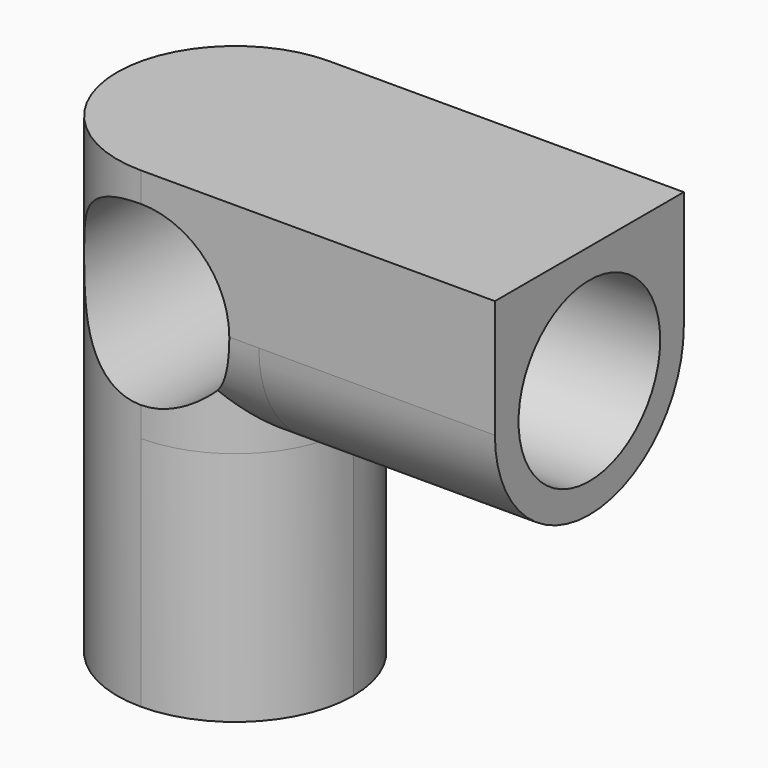
from build123d import *

# Parameters (mm, degrees)
F0_R         = 15
F1_DEPTH     = 40
F2_R         = 13
F3_DEPTH     = 40
F4_R         = 15
F5_DEPTH     = 40
F6_T3_DEPTH  = 40
F6_T6_DEPTH  = 40
F6_T9_DEPTH  = 80
F6_T12_DEPTH = 80
F6_T15_DEPTH = 40
F6_T18_DEPTH = 40
F6_T22_DEPTH = 90
F6_T26_DEPTH = 90
F6_T32_DEPTH = 90
F6_T36_DEPTH = 90


# Not quite as in the source:
# - a fillet or chamfer that OpenCascade refuses, or shapes differently, is made with other operations: its cross-section is extruded or revolved along the edge and cut away or added
# - a feature of the source that left no trace in its solid (it failed there, or was rolled back) is left out


with BuildPart() as f1:
    # F0 (on Front) → F1 (new body)
    with BuildSketch(Plane.XZ):
        Polygon((15, -40.7675257325), (15, -0.7675257325), (55, -0.7675257325), (55, 39.2324742675), (-25, 39.2324742675), (-25, -40.7675257325), align=None)
        with Locations((-5, 19.2324742675)):
            Circle(F0_R, mode=Mode.SUBTRACT)
    extrude(amount=F1_DEPTH)

    # F2 (on face) → F3 (cut)
    with BuildSketch(Plane(origin=(0, 0, -40.7675257325), x_dir=(1, 0, 0), z_dir=(0, 0, -1))):
        with Locations((-5, 20)):
            Circle(F2_R)
    extrude(amount=-F3_DEPTH, mode=Mode.SUBTRACT)

    # F4 (on face) → F5 (cut)
    with BuildSketch(Plane.YZ.offset(55)):
        with Locations((-20, 19.2324742675)):
            Circle(F4_R)
    extrude(amount=-F5_DEPTH, mode=Mode.SUBTRACT)

    # F6: fillet of radius 20 on 6 edges, made by hand


with BuildPart() as f6_tool1:
    # F6_s2 → F6_t3 (new body)
    with BuildSketch(Plane.XY.offset(-40.7675257325)):
        with BuildLine():
            ThreePointArc((-5, 0), (9.1421356237, -5.8578643763), (15, -20))
            Line((15, -20), (15.4, -20))
            Line((15.4, -20), (15.4, 0.4))
            Line((15.4, 0.4), (-5, 0.4))
            Line((-5, 0.4), (-5, 0))
        make_face()
    extrude(amount=F6_T3_DEPTH)


with BuildPart() as f6_tool4:
    # F6_s5 → F6_t6 (new body)
    with BuildSketch(Plane.XY.offset(-40.7675257325)):
        with BuildLine():
            ThreePointArc((-5, -40), (9.1421356237, -34.1421356237), (15, -20))
            Line((15, -20), (15.4, -20))
            Line((15.4, -20), (15.4, -40.4))
            Line((15.4, -40.4), (-5, -40.4))
            Line((-5, -40.4), (-5, -40))
        make_face()
    extrude(amount=F6_T6_DEPTH)


with BuildPart() as f6_tool7:
    # F6_s8 → F6_t9 (new body)
    with BuildSketch(Plane.XY.offset(39.2324742675)):
        with BuildLine():
            ThreePointArc((-25, -20), (-19.1421356237, -34.1421356237), (-5, -40))
            Line((-5, -40), (-5, -40.4))
            Line((-5, -40.4), (-25.4, -40.4))
            Line((-25.4, -40.4), (-25.4, -20))
            Line((-25.4, -20), (-25, -20))
        make_face()
    extrude(amount=-F6_T9_DEPTH)


with BuildPart() as f6_tool10:
    # F6_s11 → F6_t12 (new body)
    with BuildSketch(Plane.XY.offset(39.2324742675)):
        with BuildLine():
            ThreePointArc((-25, -20), (-19.1421356237, -5.8578643763), (-5, 0))
            Line((-5, 0), (-5, 0.4))
            Line((-5, 0.4), (-25.4, 0.4))
            Line((-25.4, 0.4), (-25.4, -20))
            Line((-25.4, -20), (-25, -20))
        make_face()
    extrude(amount=-F6_T12_DEPTH)


with BuildPart() as f6_tool13:
    # F6_s14 → F6_t15 (new body)
    with BuildSketch(Plane.YZ.offset(15)):
        with BuildLine():
            ThreePointArc((0, 19.2324742675), (-5.8578643763, 5.0903386438), (-20, -0.7675257325))
            Line((-20, -0.7675257325), (-20, -1.1675257325))
            Line((-20, -1.1675257325), (0.4, -1.1675257325))
            Line((0.4, -1.1675257325), (0.4, 19.2324742675))
            Line((0.4, 19.2324742675), (0, 19.2324742675))
        make_face()
    extrude(amount=F6_T15_DEPTH)


with BuildPart() as f6_tool16:
    # F6_s17 → F6_t18 (new body)
    with BuildSketch(Plane.YZ.offset(15)):
        with BuildLine():
            ThreePointArc((-40, 19.2324742675), (-34.1421356237, 5.0903386438), (-20, -0.7675257325))
            Line((-20, -0.7675257325), (-20, -1.1675257325))
            Line((-20, -1.1675257325), (-40.4, -1.1675257325))
            Line((-40.4, -1.1675257325), (-40.4, 19.2324742675))
            Line((-40.4, 19.2324742675), (-40, 19.2324742675))
        make_face()
    extrude(amount=F6_T18_DEPTH)


with BuildPart() as f6_tool20:
    # F6_s21 → F6_t22 (new body)
    with BuildSketch(Plane.XY.offset(-40.7675257325)):
        with BuildLine():
            ThreePointArc((-5, 0), (9.1421356237, -5.8578643763), (15, -20))
            Line((15, -20), (15.4, -20))
            Line((15.4, -20), (15.4, 0.4))
            Line((15.4, 0.4), (-5, 0.4))
            Line((-5, 0.4), (-5, 0))
        make_face()
    extrude(amount=F6_T22_DEPTH)

    split(bisect_by=Plane.XY.offset(-0.7675257325), keep=Keep.TOP)


with BuildPart() as f6_tool24:
    # F6_s25 → F6_t26 (new body)
    with BuildSketch(Plane.YZ.offset(-35)):
        with BuildLine():
            ThreePointArc((0, 19.2324742675), (-5.8578643763, 5.0903386438), (-20, -0.7675257325))
            Line((-20, -0.7675257325), (-20, -1.1675257325))
            Line((-20, -1.1675257325), (0.4, -1.1675257325))
            Line((0.4, -1.1675257325), (0.4, 19.2324742675))
            Line((0.4, 19.2324742675), (0, 19.2324742675))
        make_face()
    extrude(amount=F6_T26_DEPTH)

    split(bisect_by=Plane.YZ.offset(15), keep=Keep.BOTTOM)


with BuildPart() as f6_tool20_1:
    add(f6_tool20.part)

    # F6_t28: intersect F6_tool24
    add(f6_tool24.part, mode=Mode.INTERSECT)


with BuildPart() as f6_tool30:
    # F6_s31 → F6_t32 (new body)
    with BuildSketch(Plane.XY.offset(-40.7675257325)):
        with BuildLine():
            ThreePointArc((-5, -40), (9.1421356237, -34.1421356237), (15, -20))
            Line((15, -20), (15.4, -20))
            Line((15.4, -20), (15.4, -40.4))
            Line((15.4, -40.4), (-5, -40.4))
            Line((-5, -40.4), (-5, -40))
        make_face()
    extrude(amount=F6_T32_DEPTH)

    split(bisect_by=Plane.XY.offset(-0.7675257325), keep=Keep.TOP)


with BuildPart() as f6_tool34:
    # F6_s35 → F6_t36 (new body)
    with BuildSketch(Plane.YZ.offset(-35)):
        with BuildLine():
            ThreePointArc((-40, 19.2324742675), (-34.1421356237, 5.0903386438), (-20, -0.7675257325))
            Line((-20, -0.7675257325), (-20, -1.1675257325))
            Line((-20, -1.1675257325), (-40.4, -1.1675257325))
            Line((-40.4, -1.1675257325), (-40.4, 19.2324742675))
            Line((-40.4, 19.2324742675), (-40, 19.2324742675))
        make_face()
    extrude(amount=F6_T36_DEPTH)

    split(bisect_by=Plane.YZ.offset(15), keep=Keep.BOTTOM)


with BuildPart() as f6_tool30_1:
    add(f6_tool30.part)

    # F6_t38: intersect F6_tool34
    add(f6_tool34.part, mode=Mode.INTERSECT)


with BuildPart() as f1_1:
    add(f1.part)

    # F6_t39: cut F6_tool1, F6_tool4, F6_tool7, F6_tool10, F6_tool13, F6_tool16, F6_tool20, F6_tool30
    add([f6_tool1.part, f6_tool4.part, f6_tool7.part, f6_tool10.part, f6_tool13.part, f6_tool16.part, f6_tool20_1.part, f6_tool30_1.part], mode=Mode.SUBTRACT)


solid = f1_1.part
